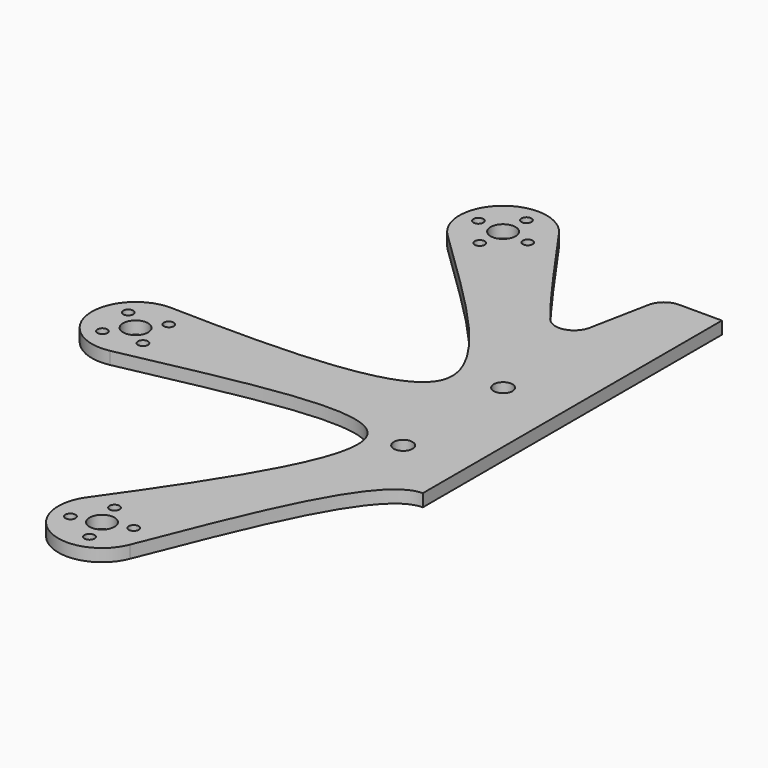
from build123d import *

# Parameters (mm, degrees)
F0_R     = 0.8
F0_R_2   = 2
F0_R_3   = 1.5
F1_DEPTH = 2


with BuildPart() as f1:
    # F0 (on Top) → F1 (new body)
    with BuildSketch(Plane.XY):
        with BuildLine():
            add(Edge.make_bspline(
                [(-30.7139102544, 47.0701435694), (-26.0563740938, 40.5834526545), (-21.5054762535, 33.727348901), (-16.9553515314, 28.1144111899)],
                knots=[0, 0, 0, 0, 0.2252580977, 0.2252580977, 0.2252580977, 0.2252580977], degree=3))
            ThreePointArc((-30.7139102544, 47.0701435694), (-40.9618832344, 48.2968026675), (-41.2923553235, 37.980968676))
            add(Edge.make_bspline(
                [(-41.2923553235, 37.980968676), (-28.2909487562, 25.2759386837), (-1.3386977002, 0.9389418911), (-37.9847105167, 0.5142288136), (-55.8291501073, 0.959428143)],
                knots=[0, 0, 0, 0, 0.5008389877, 1, 1, 1, 1], degree=3))
            ThreePointArc((-55.8291501073, 0.959428143), (-62.9764861299, -6.6554726404), (-54.6028941093, -12.8967932407))
            add(Edge.make_bspline(
                [(-54.6028941093, -12.8967932407), (-36.6411490662, -9.2280647487), (-1.5554346637, -0.6002486072), (-21.8125444782, -31.161686503), (-32.1135049914, -45.7143883537)],
                knots=[0, 0, 0, 0, 0.5007521355, 1, 1, 1, 1], degree=3))
            ThreePointArc((-32.1135049914, -45.7143883537), (-29.7366902879, -55.9122023453), (-19.8935436127, -52.3404910086))
            add(Edge.make_bspline(
                [(-19.8935436127, -52.3404910086), (-13.1991680642, -35.4702565974), (-6.6281586733, -18.5581652323), (0, -18.5741237139)],
                knots=[0, 0, 0, 0, 0.5001011209, 0.5001011209, 0.5001011209, 0.5001011209], degree=3))
            Line((0, -18.5741237139), (0, 16.0465487335))
            add(Edge.make_bspline(
                [(-16.9553515314, 28.1144111899), (-11.3677507043, 21.221664878), (-5.7813157469, 16.2036250536), (0, 16.0465487335)],
                knots=[0.2252580977, 0.2252580977, 0.2252580977, 0.2252580977, 0.5018774016, 0.5018774016, 0.5018774016, 0.5018774016], degree=3))
        make_face()
        with Locations((-30.4631808179, -51.0048452558)):
            Circle(F0_R, mode=Mode.SUBTRACT)
        with Locations((-25.1537810623, -53.821807136)):
            Circle(F0_R, mode=Mode.SUBTRACT)
        with Locations((-26.4, -49.7586263181)):
            Circle(F0_R_2, mode=Mode.SUBTRACT)
        with Locations((-27.6462189377, -45.6954455001)):
            Circle(F0_R, mode=Mode.SUBTRACT)
        with Locations((-22.3368191821, -48.5124073803)):
            Circle(F0_R, mode=Mode.SUBTRACT)
        with Locations((-58.6694667332, -9.3484382842)):
            Circle(F0_R, mode=Mode.SUBTRACT)
        with Locations((-52.6936941752, -8.7041228837)):
            Circle(F0_R, mode=Mode.SUBTRACT)
        with Locations((-56.0037381545, -6.038394305)):
            Circle(F0_R_2, mode=Mode.SUBTRACT)
        with Locations((-10, -10)):
            Circle(F0_R_3, mode=Mode.SUBTRACT)
        with Locations((-59.3137821338, -3.3726657263)):
            Circle(F0_R, mode=Mode.SUBTRACT)
        with Locations((-53.3380095758, -2.7283503257)):
            Circle(F0_R, mode=Mode.SUBTRACT)
        with Locations((-10, 10)):
            Circle(F0_R_3, mode=Mode.SUBTRACT)
        with Locations((-36.7514506951, 38.752006823)):
            Circle(F0_R, mode=Mode.SUBTRACT)
        with Locations((-40.6354435906, 43.3389011087)):
            Circle(F0_R, mode=Mode.SUBTRACT)
        with Locations((-36.4, 42.9874504136)):
            Circle(F0_R_2, mode=Mode.SUBTRACT)
        with Locations((-32.1645564094, 42.6359997185)):
            Circle(F0_R, mode=Mode.SUBTRACT)
        with Locations((-36.0485493049, 47.2228940042)):
            Circle(F0_R, mode=Mode.SUBTRACT)
        with BuildLine():
            ThreePointArc((-11.6817113012, 29.4225234538), (-13.9026459734, 27.0918297248), (-16.9553515314, 28.1144111899))
            add(Edge.make_bspline(
                [(-16.9553515314, 28.1144111899), (-11.3677507043, 21.221664878), (-5.7813157469, 16.2036250536), (0, 16.0465487335)],
                knots=[0.2252580977, 0.2252580977, 0.2252580977, 0.2252580977, 0.5018774016, 0.5018774016, 0.5018774016, 0.5018774016], degree=3))
            Line((0, 16.0465487335), (0, 41.2778827355))
            Line((0, 41.2778827355), (-6.8755115637, 41.2778827355))
            ThreePointArc((-6.8755115637, 41.2778827355), (-8.7803475094, 40.5955539849), (-9.8187005677, 38.8589494156))
            Line((-9.8187005677, 38.8589494156), (-11.6817113012, 29.4225234538))
        make_face()
    extrude(amount=F1_DEPTH)


solid = f1.part
